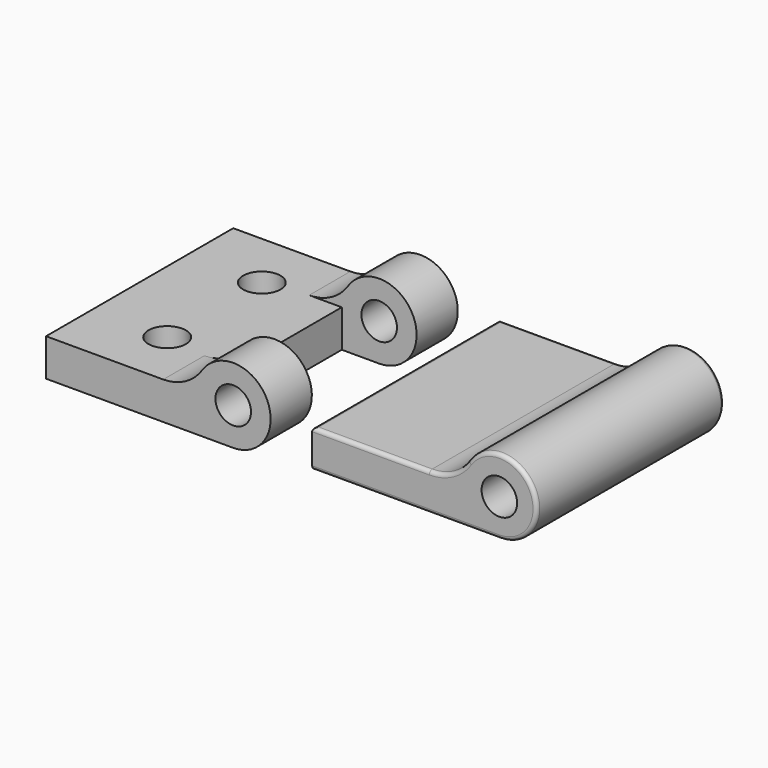
from build123d import *

# Parameters (mm, degrees)
F0_R          = 2.413
F1_DEPTH      = 31.75
F2_W          = 10.16
F2_H          = 17.78
F3_DEPTH      = 5.08
F3_DEPTH_BACK = 107
F4_R          = 2.54
F5_DEPTH      = 5.08
F6_R          = 6.35
F6_2_R        = 6.35
F7_R          = 0.508


# Not quite as in the source:
# - an extrude ends at something that could not be found from the text; its depth is read off the source's solid


with BuildPart() as f1:
    # F0 (on Front) → F1 (new body)
    with BuildSketch(Plane.XZ):
        with BuildLine():
            Line((-41.1975002551, 5.7546137058), (-61.5175002551, 5.7546137058))
            Line((-61.5175002551, 5.7546137058), (-61.5175002551, 0.6746137058))
            Line((-61.5175002551, 0.6746137058), (-36.1175002551, 0.6746137058))
            ThreePointArc((-36.1175002551, 0.6746137058), (-32.5253978067, 9.3467161542), (-41.1975002551, 5.7546137058))
        make_face()
        with Locations((-36.1175002551, 5.7546137058)):
            Circle(F0_R, mode=Mode.SUBTRACT)
    extrude(amount=F1_DEPTH)

    # F2 (on face) → F3 (cut, two sides)
    with BuildSketch(Plane.XY.offset(5.7546137058)) as f3_sk:
        with Locations((-36.1175002551, -15.875)):
            Rectangle(F2_W, F2_H)
    extrude(amount=-F3_DEPTH, mode=Mode.SUBTRACT)
    extrude(f3_sk.sketch, amount=F3_DEPTH_BACK, mode=Mode.SUBTRACT)

    # F4 (on face) → F5 (cut, through all)
    with BuildSketch(Plane.XY.offset(5.7546137058)):
        with Locations((-51.3575002551, -7.8484792235)):
            Circle(F4_R)
        with Locations((-51.3575002551, -23.9015207765)):
            Circle(F4_R)
    extrude(amount=-F5_DEPTH, mode=Mode.SUBTRACT)

    # F6#2
    f6_2_edges = [f1.edges().sort_by_distance(p)[0] for p in [
        (-41.1975, -3.4925, 5.754614),
        (-41.1975, -28.2575, 5.754614),
    ]]
    fillet(f6_2_edges, radius=F6_2_R)


with BuildPart() as f1b:
    # F0 (on Front) → F1, piece 2 (new body)
    with BuildSketch(Plane.XZ):
        with BuildLine():
            Line((-5.08, 6.5988614224), (-25.4, 6.5988614224))
            Line((-25.4, 6.5988614224), (-25.4, 1.5188614224))
            Line((-25.4, 1.5188614224), (0, 1.5188614224))
            ThreePointArc((0, 1.5188614224), (3.5921024484, 10.1909638708), (-5.08, 6.5988614224))
        make_face()
        with Locations((0, 6.5988614224)):
            Circle(F0_R, mode=Mode.SUBTRACT)
    extrude(amount=F1_DEPTH)

    # F6
    f6_edges = [f1b.edges().sort_by_distance(p)[0] for p in [
        (-5.08, -15.875, 6.598861),
    ]]
    fillet(f6_edges, radius=F6_R)

    # F7
    f7_edges = [f1b.edges().sort_by_distance(p)[0] for p in [
        (-17.451905, -31.75, 6.598861),
        (-17.451905, 0, 6.598861),
        (-25.4, -15.875, 6.598861),
        (4.480139, 0, 8.993596),
        (4.480139, -31.75, 8.993596),
        (-6.510391, 0, 7.348688),
        (-12.7, 0, 1.518861),
        (-6.510391, -31.75, 7.348688),
        (-12.7, -31.75, 1.518861),
    ]]
    fillet(f7_edges, radius=F7_R)


solid = Compound([f1.part, f1b.part])
